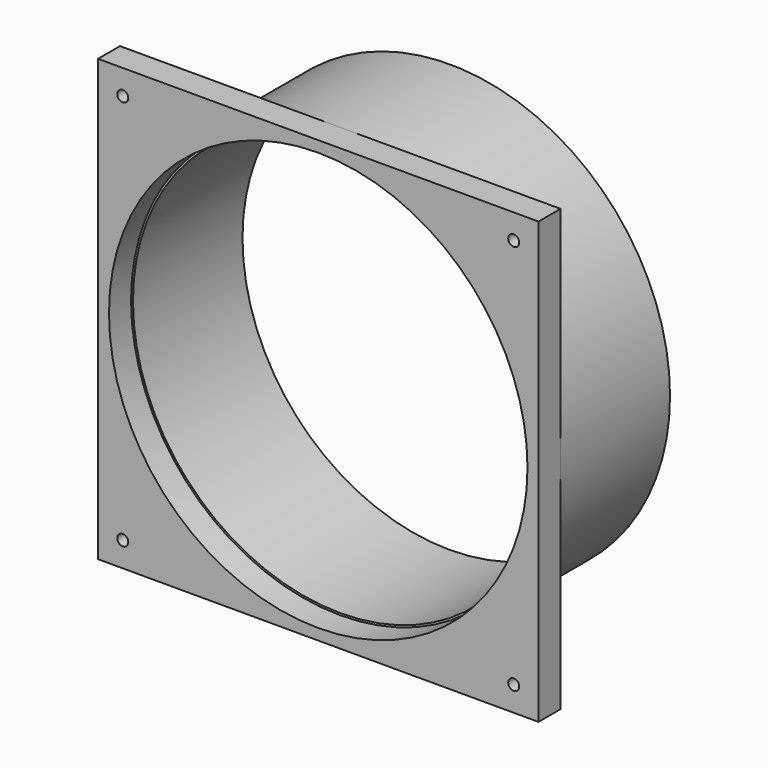
from build123d import *

# Parameters (mm, degrees)
F0_W     = 80
F0_H     = 80
F0_R     = 1
F0_R_2   = 38
F1_DEPTH = 2.5
F3_R     = 40
F3_R_2   = 37.6432669416
F4_DEPTH = 24.8567536473


with BuildPart() as f1:
    # F0 (on Front) → F1 (new body, symmetric)
    with BuildSketch(Plane.XZ):
        Rectangle(F0_W, F0_H)
        with Locations((-35.5, -35.5)):
            Circle(F0_R, mode=Mode.SUBTRACT)
        with Locations((35.5, -35.5)):
            Circle(F0_R, mode=Mode.SUBTRACT)
        with Locations((-35.5, 35.5)):
            Circle(F0_R, mode=Mode.SUBTRACT)
        Circle(F0_R_2, mode=Mode.SUBTRACT)
        with Locations((35.5, 35.5)):
            Circle(F0_R, mode=Mode.SUBTRACT)
    extrude(amount=F1_DEPTH, both=True)

    # F3 (on face) → F4 (join)
    with BuildSketch(Plane(origin=(0, 2.5, 0), x_dir=(-1, 0, 0), z_dir=(0, 1, 0))):
        Circle(F3_R)
        Circle(F3_R_2, mode=Mode.SUBTRACT)
    extrude(amount=F4_DEPTH)


solid = f1.part
